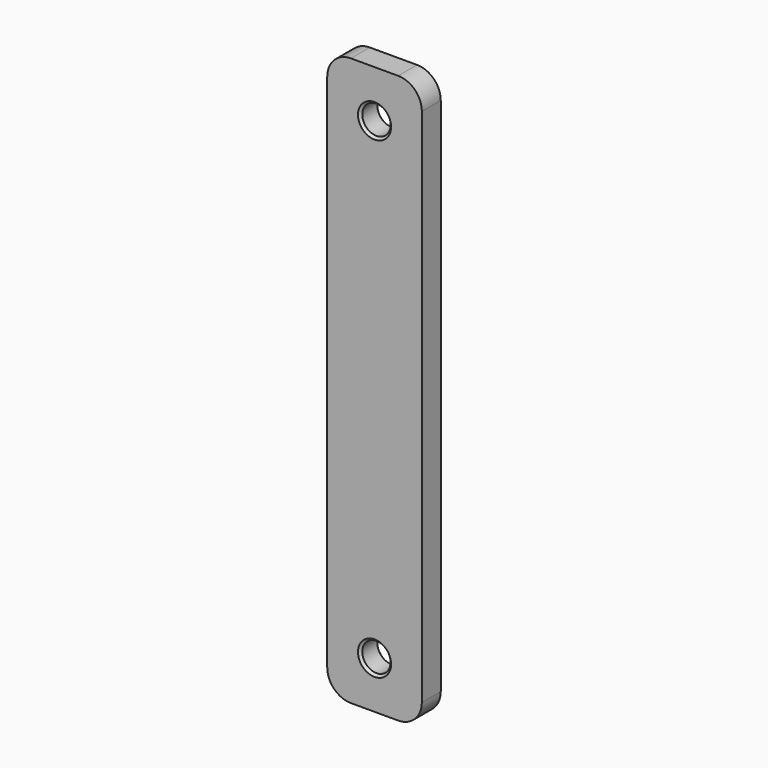
from build123d import *

# Parameters (mm, degrees)
F0_W     = 20
F0_H     = 120
F1_DEPTH = 5
F2_R     = 3
F3_DEPTH = 5.001
F5_D     = 6
F6_SIZE  = 0.5
F7_R     = 5


with BuildPart() as f1:
    # F0 (on Front) → F1 (new body)
    with BuildSketch(Plane.XZ):
        with Locations((10, 60)):
            Rectangle(F0_W, F0_H)
    extrude(amount=F1_DEPTH)

    # F2 (on face) → F3 (cut, through all)
    with BuildSketch(Plane.XZ.offset(5)):
        with Locations((10, 110)):
            Circle(F2_R)
    extrude(amount=-F3_DEPTH, mode=Mode.SUBTRACT)

    # F5 (through all)
    with Locations(Plane.XZ.offset(5)):
        with Locations((10, 10)):
            Hole(F5_D / 2)

    # F6
    f6_edges = [f1.edges().sort_by_distance(p)[0] for p in [
        (7, -5, 110),
        (7, 0, 110),
        (7, 0, 10),
        (7, -5, 10),
    ]]
    chamfer(f6_edges, length=F6_SIZE)

    # F7
    f7_edges = [f1.edges().sort_by_distance(p)[0] for p in [
        (20, -2.5, 120),
        (0, -2.5, 120),
        (20, -2.5, 0),
        (0, -2.5, 0),
    ]]
    fillet(f7_edges, radius=F7_R)


solid = f1.part
